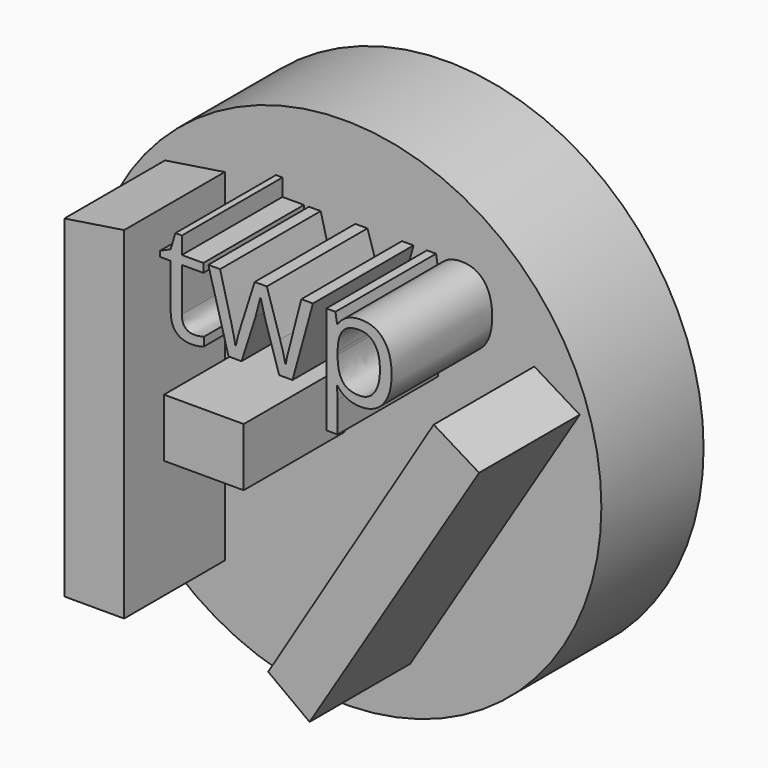
from build123d import *

# Parameters (mm, degrees)
F0_R         = 51.1098270936
F1_DEPTH     = 25.4
F2_W         = 15.8413928002
F2_H         = 11.585084023
F3_DEPTH     = 25
F4_TEXT_SIZE = 27.5174880193
F5_DEPTH     = 25


# Not quite as in the source:
# - Text() gives the source's letters only with a copy of the font that has no kerning and outlines rounded to 1/6400 em; it was checked with that copy


with BuildPart() as f1:
    # F0 (on Front) → F1 (new body)
    with BuildSketch(Plane.XZ):
        Circle(F0_R)
    extrude(amount=F1_DEPTH)

    # F2 (on face) → F3 (join)
    with BuildSketch(Plane.XZ.offset(25.4)):
        Polygon((-23.7620901316, 34.282296896), (-35.6431342661, 32.453071326), (-35.6431342661, -33.7038598955), (-23.7620901316, -33.7038598955), align=None)
        with Locations((-7.9206964001, 2.2708786419)):
            Rectangle(F2_W, F2_H)
        Polygon((37.775631994, 20.2582478523), (4.8742755316, -33.7038598955), (13.0996126682, -39.801273495), (46.8019881381, 14.7547682173), align=None)
    extrude(amount=F3_DEPTH)

    # F4 (on face) → F5 (join)
    with BuildSketch(Plane.XZ.offset(25.4)):
        with Locations((-17.0494187623, 18.9224369824)):
            Text('twp', F4_TEXT_SIZE, font='Open Sans', text_align=(TextAlign.LEFT, TextAlign.BOTTOM))
    extrude(amount=F5_DEPTH)


solid = f1.part
